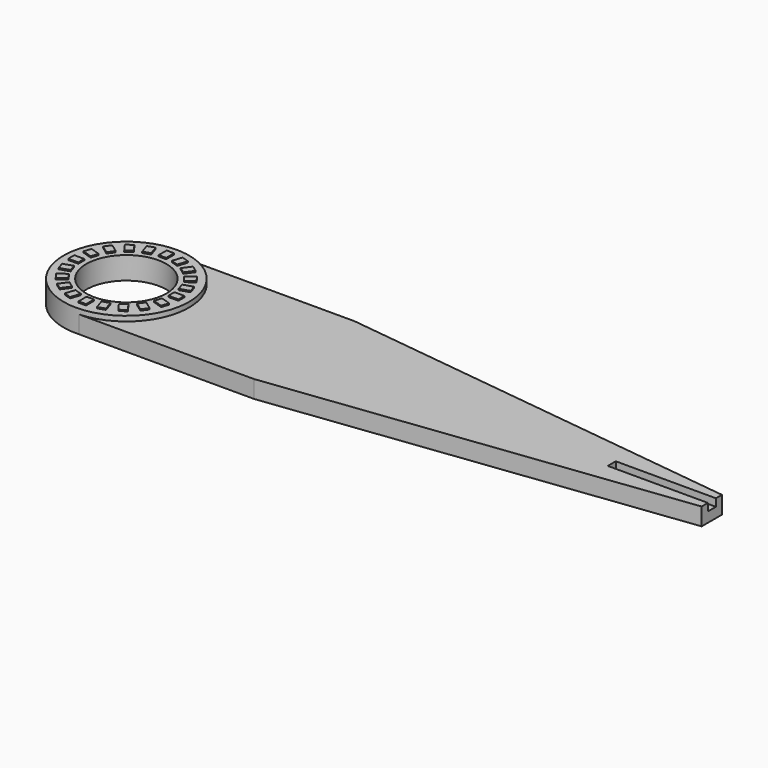
from build123d import *

# Parameters (mm, degrees)
F0_R         = 8
F1_DEPTH     = 3.5
F2_R         = 8
F3_DEPTH     = 1
F4_W         = 1.5
F4_H         = 2
F4_W_2       = 2
F4_H_2       = 1.5
F5_DEPTH     = 0.25
F6_W         = 20
F6_H         = 2
F7_DEPTH     = 1.5
F9_TEXT_SIZE = 15.2773784108
F10_DEPTH    = 1


# Not quite as in the source:
# - Text() gives the source's letters only with a copy of the font that has no kerning and outlines rounded to 1/6400 em; it was checked with that copy


with BuildPart() as f1:
    # F0 (on Top) → F1 (new body)
    with BuildSketch(Plane.XY):
        with BuildLine():
            Line((116.9446667232, 2.5315263231), (35.5558822886, 12.5248124823))
            Line((35.5558822886, 12.5248124823), (0.5558822886, 12.5248124823))
            ThreePointArc((0.5558822886, 12.5248124823), (-12.5371421319, 0), (0.5558822886, -12.5248124823))
            Line((0.5558822886, -12.5248124823), (35.5558822886, -12.5248124823))
            Line((35.5558822886, -12.5248124823), (116.9446667232, -2.5315263231))
            Line((116.9446667232, -2.5315263231), (116.9446667232, 2.5315263231))
        make_face()
        Circle(F0_R, mode=Mode.SUBTRACT)
    extrude(amount=F1_DEPTH)

    # F2 (on face) → F3 (join)
    with BuildSketch(Plane.XY.offset(3.5)):
        with BuildLine():
            ThreePointArc((0.5558822886, -12.5248124823), (9.0595007615, -8.6663359494), (12.5371421319, 0))
            ThreePointArc((12.5371421319, 0), (9.0595007615, 8.6663359494), (0.5558822886, 12.5248124823))
            ThreePointArc((0.5558822886, 12.5248124823), (-12.5371421319, 0), (0.5558822886, -12.5248124823))
        make_face()
        Circle(F2_R, mode=Mode.SUBTRACT)
    extrude(amount=F3_DEPTH)

    # F4 (on face) → F5 (join)
    with BuildSketch(Plane.XY.offset(4.5)):
        Polygon((-2.6858945509, 10.693384425), (-4.1124793253, 10.2298589335), (-3.4944453366, 8.3277459009), (-2.0678605622, 8.7912713924), align=None)
        with Locations((0, 10)):
            Rectangle(F4_W, F4_H)
        Polygon((4.1124793253, 10.2298589335), (2.6858945509, 10.693384425), (2.0678605622, 8.7912713924), (3.4944453366, 8.3277459009), align=None)
        Polygon((7.072400521, 8.4583479989), (5.8588750294, 9.3400258773), (4.6833045249, 7.7219918886), (5.8968300164, 6.8403140102), align=None)
        Polygon((9.3400258773, 5.8588750294), (8.4583479989, 7.072400521), (6.8403140102, 5.8968300164), (7.7219918886, 4.6833045249), align=None)
        Polygon((10.693384425, 2.6858945509), (10.2298589335, 4.1124793253), (8.3277459009, 3.4944453366), (8.7912713924, 2.0678605622), align=None)
        with Locations((10, 0)):
            Rectangle(F4_W_2, F4_H_2)
        Polygon((10.2298589335, -4.1124793253), (10.693384425, -2.6858945509), (8.7912713924, -2.0678605622), (8.3277459009, -3.4944453366), align=None)
        Polygon((8.4583479989, -7.072400521), (9.3400258773, -5.8588750294), (7.7219918886, -4.6833045249), (6.8403140102, -5.8968300164), align=None)
        Polygon((5.8588750294, -9.3400258773), (7.072400521, -8.4583479989), (5.8968300164, -6.8403140102), (4.6833045249, -7.7219918886), align=None)
        Polygon((2.6858945509, -10.693384425), (4.1124793253, -10.2298589335), (3.4944453366, -8.3277459009), (2.0678605622, -8.7912713924), align=None)
        with Locations((0, -10)):
            Rectangle(F4_W, F4_H)
        Polygon((-4.1124793253, -10.2298589335), (-2.6858945509, -10.693384425), (-2.0678605622, -8.7912713924), (-3.4944453366, -8.3277459009), align=None)
        Polygon((-7.072400521, -8.4583479989), (-5.8588750294, -9.3400258773), (-4.6833045249, -7.7219918886), (-5.8968300164, -6.8403140102), align=None)
        Polygon((-9.3400258773, -5.8588750294), (-8.4583479989, -7.072400521), (-6.8403140102, -5.8968300164), (-7.7219918886, -4.6833045249), align=None)
        Polygon((-10.693384425, -2.6858945509), (-10.2298589335, -4.1124793253), (-8.3277459009, -3.4944453366), (-8.7912713924, -2.0678605622), align=None)
        with Locations((-10, 0)):
            Rectangle(F4_W_2, F4_H_2)
        Polygon((-10.2298589335, 4.1124793253), (-10.693384425, 2.6858945509), (-8.7912713924, 2.0678605622), (-8.3277459009, 3.4944453366), align=None)
        Polygon((-8.4583479989, 7.072400521), (-9.3400258773, 5.8588750294), (-7.7219918886, 4.6833045249), (-6.8403140102, 5.8968300164), align=None)
        Polygon((-5.8588750294, 9.3400258773), (-7.072400521, 8.4583479989), (-5.8968300164, 6.8403140102), (-4.6833045249, 7.7219918886), align=None)
    extrude(amount=F5_DEPTH)

    # F6 (on face) → F7 (cut)
    with BuildSketch(Plane.XY.offset(3.5)):
        with Locations((106.9446667232, 0.0315263231)):
            Rectangle(F6_W, F6_H)
    extrude(amount=-F7_DEPTH, mode=Mode.SUBTRACT)

    # F9 (on line) → F10 (cut)
    with BuildSketch(Plane(origin=(0, 0, 0), x_dir=(1, 0, 0), z_dir=(0, 0, -1))):
        with Locations((12, -5.4998562279)):
            Text('Malfoy', F9_TEXT_SIZE, font='Open Sans', text_align=(TextAlign.LEFT, TextAlign.BOTTOM))
    extrude(amount=-F10_DEPTH, mode=Mode.SUBTRACT)


solid = f1.part
